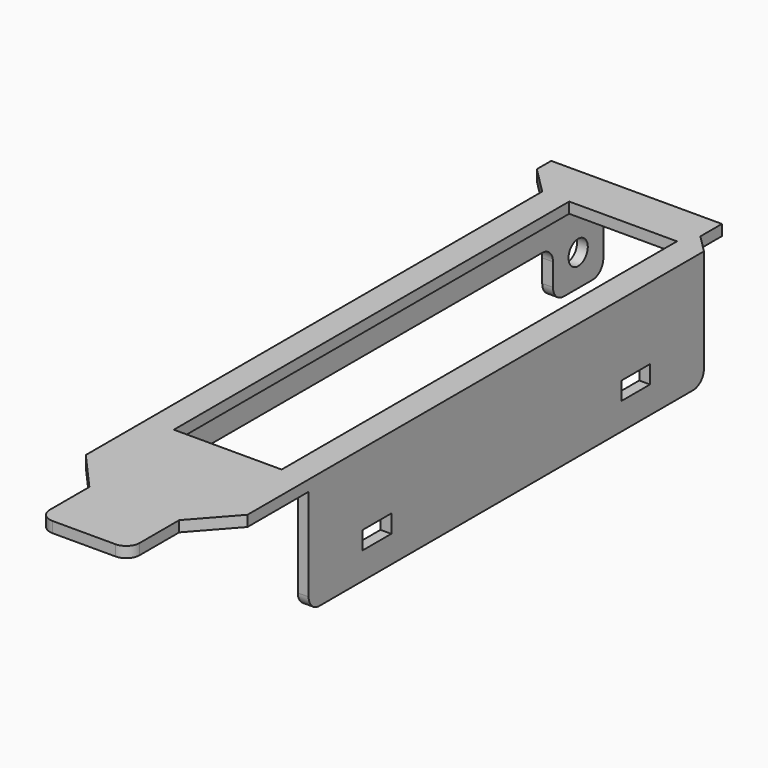
from build123d import *

# Parameters (mm, degrees)
F1_DEPTH = 1.2
F2_W     = 1.2
F2_H     = 55
F3_DEPTH = 11.8
F4_W     = 4
F4_H     = 2
F5_DEPTH = 25
F2_H_2   = 2
F6_DEPTH = 9.3
F7_W     = 55
F7_H     = 5.5
F7_R     = 1.3402800484
F8_DEPTH = 5
F11_R    = 1.5


with BuildPart() as f1:
    # F0 (on Top) → F1 (new body)
    with BuildSketch(Plane.XY):
        Polygon((0, 63.5), (0, 0), (18, 0), (18, 63.5), (15, 63.5), (15, 8.5), (3, 8.5), (3, 63.5), align=None)
        Polygon((18, 0), (0, 0), (4, -4.5), (4, -11.5), (14, -11.5), (14, -4.5), align=None)
        Polygon((-3, 66.5), (0, 63.5), (3, 63.5), (15, 63.5), (18, 63.5), (16, 65.5), (16, 68.5), (-3, 68.5), align=None)
    extrude(amount=F1_DEPTH)

    # F2 (on face) → F3 (join)
    with BuildSketch(Plane(origin=(0, 0, 0), x_dir=(1, 0, 0), z_dir=(0, 0, -1))):
        with Locations((17.4, -36)):
            Rectangle(F2_W, F2_H)
    extrude(amount=F3_DEPTH)

    # F4 (on face) → F5 (cut)
    with BuildSketch(Plane.YZ.offset(18)):
        with Locations((18, -7.8)):
            Rectangle(F4_W, F4_H)
        with Locations((54, -7.8)):
            Rectangle(F4_W, F4_H)
    extrude(amount=-F5_DEPTH, mode=Mode.SUBTRACT)

    # F2 (on face) → F6 (join)
    with BuildSketch(Plane(origin=(0, 0, 0), x_dir=(1, 0, 0), z_dir=(0, 0, -1))):
        Polygon((0, -68.5), (1.2, -68.5), (1.2, -8.5), (0, -8.5), (0, -63.5), align=None)
        with Locations((0.6, -69.5)):
            Rectangle(F2_W, F2_H_2)
    extrude(amount=F6_DEPTH)

    # F7 (on face) → F8 (cut)
    with BuildSketch(Plane(origin=(0, 0, 0), x_dir=(0, -1, 0), z_dir=(-1, 0, 0))):
        with Locations((-36, -6.55)):
            Rectangle(F7_W, F7_H)
        with Locations((-67, -5.8)):
            Circle(F7_R)
    extrude(amount=-F8_DEPTH, mode=Mode.SUBTRACT)

    # F11
    f11_edges = [f1.edges().sort_by_distance(p)[0] for p in [
        (0.6, 70.5, -9.3),
        (0.6, 63.5, -9.3),
        (0.6, 8.5, -3.8),
        (17.4, 8.5, -11.8),
        (17.4, 63.5, -11.8),
        (4, -11.5, 0.6),
        (14, -11.5, 0.6),
        (0.6, 70.5, 0),
        (0.6, 63.5, -3.8),
    ]]
    fillet(f11_edges, radius=F11_R)


solid = f1.part
